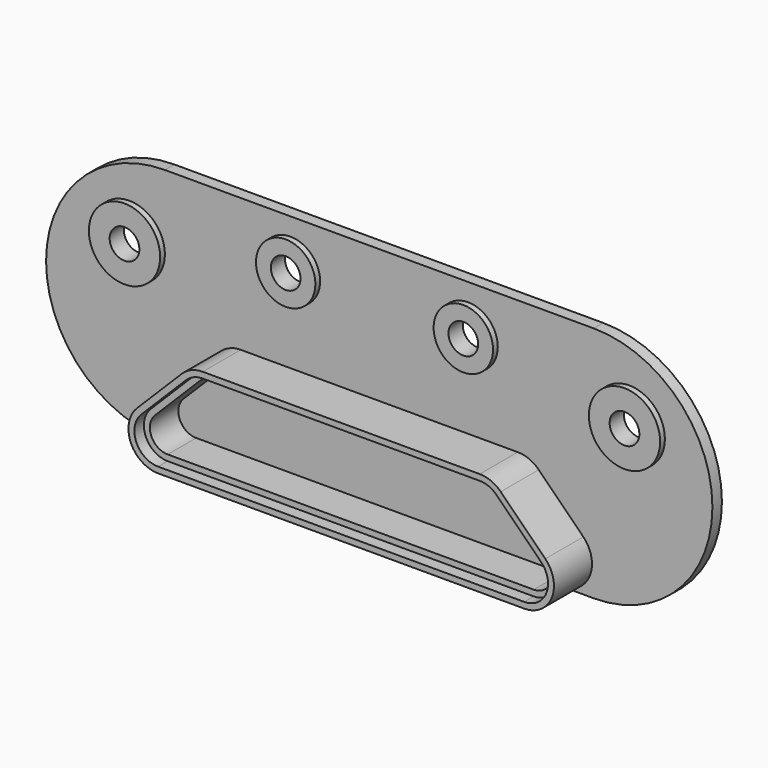
from build123d import *

# Parameters (mm, degrees)
F1_DEPTH  = 2
F3_DEPTH  = 8
F5_DEPTH  = 2
F7_DEPTH  = 6
F8_R      = 5
F8_R_2    = 6
F9_DEPTH  = 1
F10_R     = 2.5
F11_R     = 2.5
F12_DEPTH = 3.001


# Not quite as in the source:
# - a feature names something its author has since deleted; it is built from what else it names


with BuildPart() as f1:
    # F0 (on Front) → F1 (new body)
    with BuildSketch(Plane.XZ):
        with BuildLine():
            Line((-36.0815, -20), (36.0815, -20))
            ThreePointArc((36.0815, -20), (56.0815, 0), (36.0815, 20))
            Line((36.0815, 20), (-36.0815, 20))
            ThreePointArc((-36.0815, 20), (-56.0815, 0), (-36.0815, -20))
        make_face()
    extrude(amount=F1_DEPTH)

    # F2 (on face) → F3 (join)
    with BuildSketch(Plane.XZ.offset(2)):
        with BuildLine():
            Line((23.3145, -2.5), (0, -2.5))
            Line((0, -2.5), (-23.3145, -2.5))
            ThreePointArc((-23.3145, -2.5), (-25.2279171618, -2.8806023374), (-26.8500339059, -3.9644660941))
            Line((-26.8500339059, -3.9644660941), (-34.3500339059, -11.4644660941))
            ThreePointArc((-34.3500339059, -11.4644660941), (-35.4338976626, -16.9134171618), (-30.8145, -20))
            Line((-30.8145, -20), (0, -20))
            Line((0, -20), (30.8145, -20))
            ThreePointArc((30.8145, -20), (35.4338976626, -16.9134171618), (34.3500339059, -11.4644660941))
            Line((34.3500339059, -11.4644660941), (26.8500339059, -3.9644660941))
            ThreePointArc((26.8500339059, -3.9644660941), (25.2279171618, -2.8806023374), (23.3145, -2.5))
        make_face()
    extrude(amount=F3_DEPTH)

    # F4 (on face) → F5 (cut)
    with BuildSketch(Plane.XZ.offset(10)):
        with BuildLine():
            Line((-26.1429271247, -4.6715728753), (-33.6429271247, -12.1715728753))
            ThreePointArc((-33.6429271247, -12.1715728753), (-34.51001813, -16.5307337295), (-30.8145, -19))
            Line((-30.8145, -19), (30.8145, -19))
            ThreePointArc((30.8145, -19), (34.51001813, -16.5307337295), (33.6429271247, -12.1715728753))
            Line((33.6429271247, -12.1715728753), (26.1429271247, -4.6715728753))
            ThreePointArc((26.1429271247, -4.6715728753), (24.8452337295, -3.80448187), (23.3145, -3.5))
            Line((23.3145, -3.5), (-23.3145, -3.5))
            ThreePointArc((-23.3145, -3.5), (-24.8452337295, -3.80448187), (-26.1429271247, -4.6715728753))
        make_face()
    extrude(amount=-F5_DEPTH, mode=Mode.SUBTRACT)

    # F6 (on face) → F7 (cut)
    with BuildSketch(Plane.XZ.offset(8)):
        with BuildLine():
            ThreePointArc((30.8145, -18), (33.5861385975, -16.1480502971), (32.9358203436, -12.8786796564))
            Line((32.9358203436, -12.8786796564), (25.4358203436, -5.3786796564))
            ThreePointArc((25.4358203436, -5.3786796564), (24.4625502971, -4.7283614025), (23.3145, -4.5))
            Line((23.3145, -4.5), (-23.3145, -4.5))
            ThreePointArc((-23.3145, -4.5), (-24.4625502971, -4.7283614025), (-25.4358203436, -5.3786796564))
            Line((-25.4358203436, -5.3786796564), (-32.9358203436, -12.8786796564))
            ThreePointArc((-32.9358203436, -12.8786796564), (-33.5861385975, -16.1480502971), (-30.8145, -18))
            Line((-30.8145, -18), (30.8145, -18))
        make_face()
    extrude(amount=-F7_DEPTH, mode=Mode.SUBTRACT)

    # F8 (on face) → F9 (join)
    with BuildSketch(Plane.XZ.offset(2)):
        with Locations((-14.952, 12)):
            Circle(F8_R)
        with Locations((-42.0815, 7.5)):
            Circle(F8_R_2)
        with Locations((14.952, 12)):
            Circle(F8_R)
        with Locations((42.0815, 7.5)):
            Circle(F8_R_2)
    extrude(amount=F9_DEPTH)

    # F10 (on face) + F11 (on face) → F12 (cut, through all)
    with BuildSketch(Plane.XZ.offset(3)):
        with Locations((-14.952, 12)):
            Circle(F10_R)
        with Locations((14.952, 12)):
            Circle(F10_R)
    with BuildSketch(Plane.XZ.offset(3)):
        with Locations((-42.0815, 7.5)):
            Circle(F11_R)
        with Locations((42.0815, 7.5)):
            Circle(F11_R)
    extrude(amount=-F12_DEPTH, mode=Mode.SUBTRACT)


solid = f1.part
